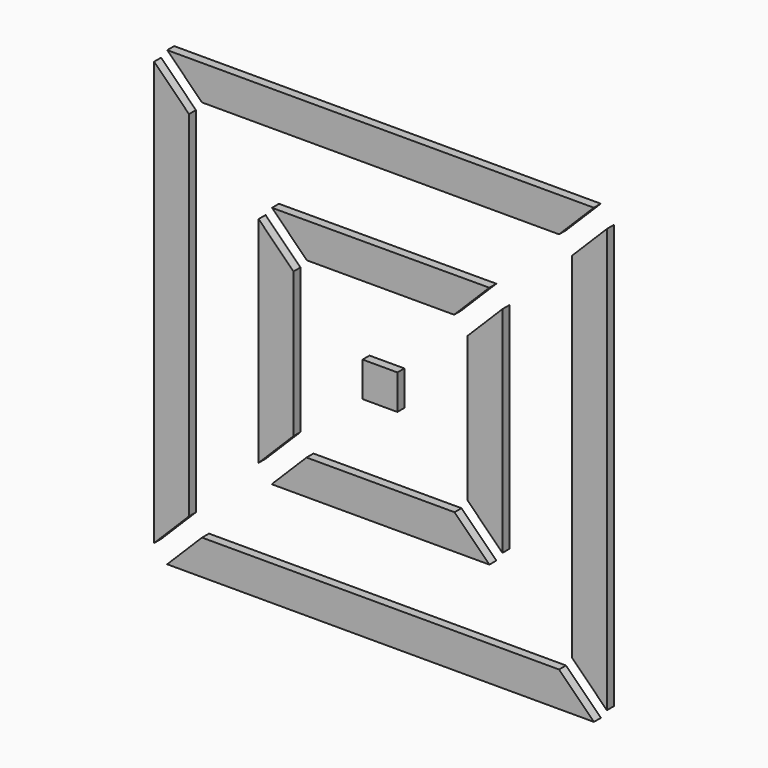
from build123d import *

# Parameters (mm, degrees)
F1_DEPTH = 25.4


with BuildPart() as f1:
    # F0 (on Front) → F1 (new body)
    with BuildSketch(Plane.XZ):
        Polygon((1217.7658302538, -186.2069594315), (1319.3658302538, -186.2069594315), (1319.3658302538, -84.6069594315), (1268.5658302538, -84.6069594315), (1268.5658302538, -135.4069594315), (1217.7658302538, -135.4069594315), align=None)
        Polygon((1268.5658302538, -84.6069594315), (1217.7658302538, -84.6069594315), (1217.7658302538, -84.6383770839), (1217.7658302538, -135.4069594315), (1268.5658302538, -135.4069594315), align=None)
    extrude(amount=F1_DEPTH)


with BuildPart() as f1b:
    # F0 (on Front) → F1, piece 2 (new body)
    with BuildSketch(Plane.XZ):
        Polygon((953.5223343681, 219.2484295396), (1055.429416395, 117.3908703306), (1484.8362563349, 117.3908703306), (1587.6884086575, 220.1930405685), align=None)
    extrude(amount=F1_DEPTH)


with BuildPart() as f1c:
    # F0 (on Front) → F1, piece 3 (new body)
    with BuildSketch(Plane.XZ):
        Polygon((1016.132836365, 63.2760249292), (1016.132836365, 75.9871864359), (914.532836365, 177.6764784897), (914.532836365, 169.5246078354), (914.532836365, -135.4069594315), (914.532836365, -448.4903973526), (1016.132836365, -346.8011052989), (1016.132836365, -135.4069594315), align=None)
    extrude(amount=F1_DEPTH)


with BuildPart() as f1d:
    # F0 (on Front) → F1, piece 4 (new body)
    with BuildSketch(Plane.XZ):
        Polygon((647.8175146307, 524.8046888061), (749.2784688856, 423.3930405685), (753.6708143363, 423.3930405685), (1270.132836365, 423.3930405685), (1786.5948583937, 423.3930405685), (1790.9872038444, 423.3930405685), (1892.4481580993, 524.8046888061), align=None)
    extrude(amount=F1_DEPTH)


with BuildPart() as f1e:
    # F0 (on Front) → F1, piece 5 (new body)
    with BuildSketch(Plane.XZ):
        Polygon((1625.732836365, 177.6764784897), (1524.132836365, 75.9871864359), (1524.132836365, -135.4069594315), (1524.132836365, -346.8011052989), (1625.732836365, -448.4903973526), (1625.732836365, -135.4069594315), align=None)
    extrude(amount=F1_DEPTH)


with BuildPart() as f1f:
    # F0 (on Front) → F1, piece 6 (new body)
    with BuildSketch(Plane.XZ):
        Polygon((1058.7386904976, -389.4069594315), (1054.2266616658, -389.4069594315), (952.5772640724, -491.0069594315), (1270.132836365, -491.0069594315), (1587.6884086575, -491.0069594315), (1486.0390110641, -389.4069594315), (1481.5269822323, -389.4069594315), (1270.132836365, -389.4069594315), align=None)
    extrude(amount=F1_DEPTH)


with BuildPart() as f1g:
    # F0 (on Front) → F1, piece 7 (new body)
    with BuildSketch(Plane.XZ):
        Polygon((711.332836365, 368.3439010905), (711.332836365, 381.0550625972), (609.732836365, 482.744354651), (609.732836365, -135.4069594315), (609.732836365, -753.558273514), (711.332836365, -651.8689814602), (711.332836365, -135.4069594315), align=None)
    extrude(amount=F1_DEPTH)


with BuildPart() as f1h:
    # F0 (on Front) → F1, piece 8 (new body)
    with BuildSketch(Plane.XZ):
        Polygon((1930.532836365, 482.744354651), (1828.932836365, 381.0550625972), (1828.932836365, -135.4069594315), (1828.932836365, -651.8689814602), (1930.532836365, -753.558273514), (1930.532836365, -135.4069594315), align=None)
    extrude(amount=F1_DEPTH)


with BuildPart() as f1i:
    # F0 (on Front) → F1, piece 9 (new body)
    with BuildSketch(Plane.XZ):
        Polygon((753.6708143363, -694.2069594315), (749.2784688856, -694.2069594315), (647.6290712922, -795.8069594315), (1270.132836365, -795.8069594315), (1892.6366014378, -795.8069594315), (1790.9872038443, -694.2069594315), (1786.5948583937, -694.2069594315), (1270.132836365, -694.2069594315), align=None)
    extrude(amount=F1_DEPTH)


solid = Compound([f1.part, f1b.part, f1c.part, f1d.part, f1e.part, f1f.part, f1g.part, f1h.part, f1i.part])
